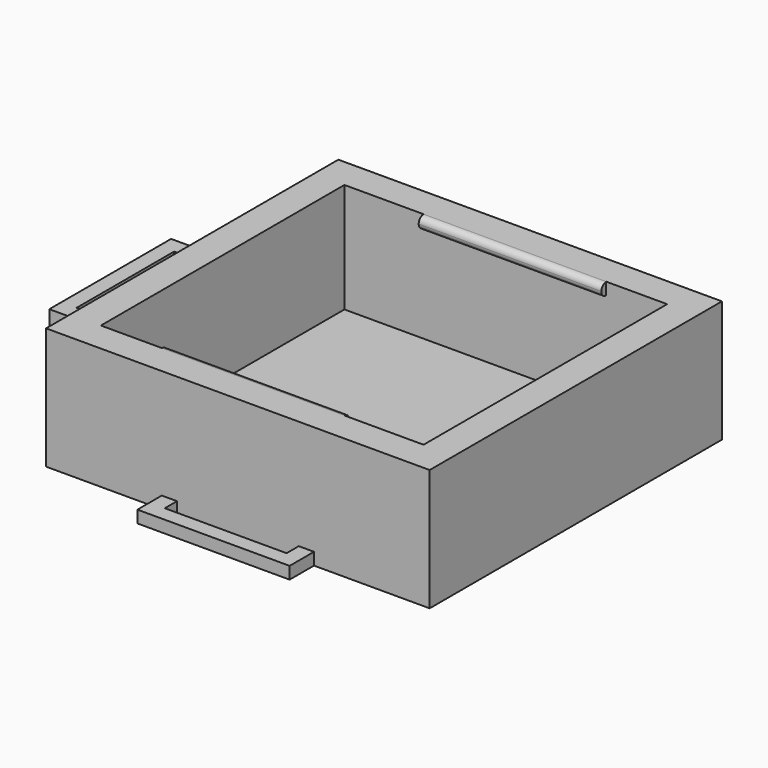
from build123d import *

# Parameters (mm, degrees)
F0_W      = 63
F0_H      = 60
F0_W_2    = 53
F0_H_2    = 50
F1_DEPTH  = 20
F3_DEPTH  = 2
F4_DEPTH  = 2
F5_W      = 30
F5_H      = 2
F6_DEPTH  = 1
F7_W      = 30
F7_H      = 2
F8_DEPTH  = 1
F9_R      = 0.99999
F10_W     = 15
F10_H     = 25
F11_DEPTH = 10
F12_W     = 12.5
F12_H     = 20
F13_DEPTH = 8
F14_R     = 2
F15_DEPTH = 25


# Not quite as in the source:
# - a fillet or chamfer is up to 0.001 mm smaller than in the source, because OpenCascade refuses the exact size


with BuildPart() as f1:
    # F0 (on Top) → F1 (new body)
    with BuildSketch(Plane.XY):
        with Locations((19.5141504109, -9.4245311618)):
            Rectangle(F0_W, F0_H)
        with Locations((19.5141504109, -9.4245311618)):
            Rectangle(F0_W_2, F0_H_2, mode=Mode.SUBTRACT)
    extrude(amount=F1_DEPTH)

    # F2 (on Top) → F3 (join)
    with BuildSketch(Plane.XY):
        Polygon((7.0141504109, 25.5754688382), (7.0141504109, 20.5754688382), (9.5141504109, 20.5754688382), (9.5141504109, 23.0754688382), (29.5141504109, 23.0754688382), (29.5141504109, 20.5754688382), (32.0141504109, 20.5754688382), (32.0141504109, 25.5754688382), align=None)
        Polygon((9.5141504109, -39.4245311618), (7.0141504109, -39.4245311618), (7.0141504109, -44.4245311618), (32.0141504109, -44.4245311618), (32.0141504109, -39.4245311618), (29.5141504109, -39.4245311618), (29.5141504109, -41.9245311618), (9.5141504109, -41.9245311618), align=None)
    extrude(amount=F3_DEPTH)

    # F0 (on Top) → F4 (join)
    with BuildSketch(Plane.XY):
        with Locations((19.5141504109, -9.4245311618)):
            Rectangle(F0_W_2, F0_H_2)
    extrude(amount=F4_DEPTH)

    # F5 (on face) → F6 (join)
    with BuildSketch(Plane.XZ.offset(-15.5754688382)):
        with Locations((21.0141504109, 19)):
            Rectangle(F5_W, F5_H)
    extrude(amount=F6_DEPTH)

    # F7 (on face) → F8 (join)
    with BuildSketch(Plane(origin=(0, -34.4245311618, 0), x_dir=(-1, 0, 0), z_dir=(0, 1, 0))):
        with Locations((-18.0141504109, 19)):
            Rectangle(F7_W, F7_H)
    extrude(amount=F8_DEPTH)

    # F9 (radius 1 in the source; OpenCascade refuses exactly that, so slightly less here)
    f9_edges = [f1.edges().sort_by_distance(p)[0] for p in [
        (21.01415, 14.575469, 20),
        (21.01415, 14.575469, 18),
        (18.01415, -33.424531, 20),
        (18.01415, -33.424531, 18),
    ]]
    fillet(f9_edges, radius=F9_R)

    # F10 (on Top) → F11 (join)
    with BuildSketch(Plane.XY):
        with Locations((-19.4858495891, -7.5094338506)):
            Rectangle(F10_W, F10_H)
    extrude(amount=F11_DEPTH)

    # F12 (on face) → F13 (cut)
    with BuildSketch(Plane.XY.offset(10)):
        with Locations((-18.2358495891, -7.5094338506)):
            Rectangle(F12_W, F12_H)
    extrude(amount=-F13_DEPTH, mode=Mode.SUBTRACT)

    # F14 (on face) → F15 (cut)
    with BuildSketch(Plane(origin=(0, 4.9905661494, 0), x_dir=(-1, 0, 0), z_dir=(0, 1, 0))):
        with Locations((19.4858495891, 6.5377363935)):
            Circle(F14_R)
    extrude(amount=-F15_DEPTH, mode=Mode.SUBTRACT)


solid = f1.part
